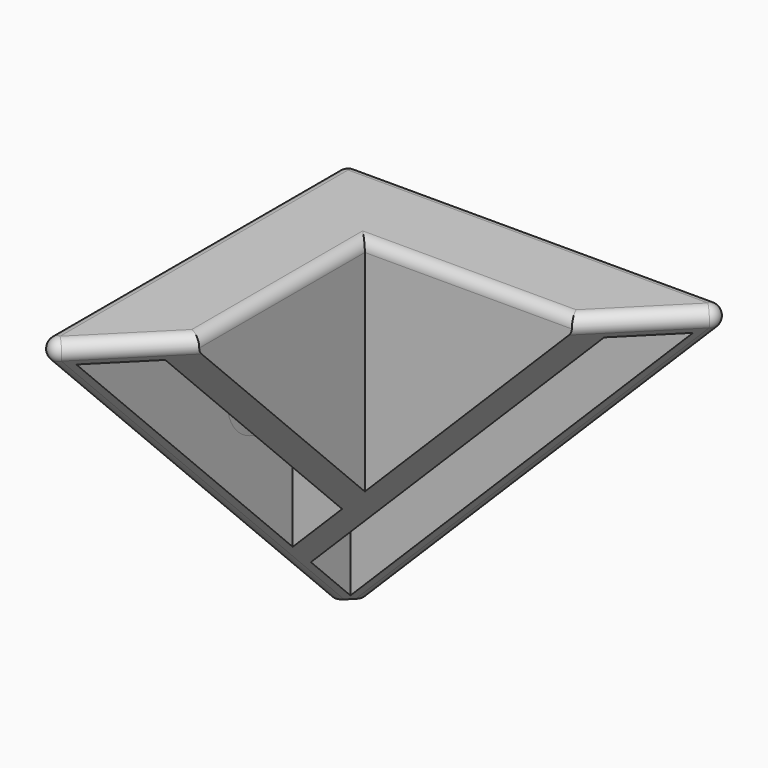
from build123d import *

# Parameters (mm, degrees)
F1_DEPTH  = 28.575
F3_R      = 38.1
F4_DEPTH  = 32.9965678842
F6_W      = 26.9748
F6_H      = 3.429
F6_W_2    = 3.429
F6_H_2    = 21.971
F7_DEPTH  = 26.9758
F14_R     = 0.762
F15_W     = 1.8396307345
F15_H     = 3.0181135691
F16_DEPTH = 26.4941772846


# Not quite as in the source:
# - a fillet or chamfer that OpenCascade refuses, or shapes differently, is made with other operations: its cross-section is extruded or revolved along the edge and cut away or added
# - a pattern or mirror of a feature is missing from the dataset's text; its kind, count and spacing are read off the source's solid


with BuildPart() as f1:
    # F0 (on Top) → F1 (new body)
    with BuildSketch(Plane.XY):
        Polygon((0, -21.971), (0, 0), (21.971, 0), (21.971, 6.604), (-6.604, 6.604), (-6.604, -21.971), align=None)
    extrude(amount=-F1_DEPTH)

    # F3 (on 3pt) → F4 (cut, through all)
    with BuildSketch(Plane(origin=(5.1223333333, -5.1223333333, -5.1223333333), x_dir=(0.4082482905, 0.8164965809, -0.4082482905), z_dir=(0.5773502692, -0.5773502692, -0.5773502692))):
        Circle(F3_R)
    extrude(amount=F4_DEPTH, mode=Mode.SUBTRACT)

    # F6 (on offset) → F7 (cut, through all)
    with BuildSketch(Plane.XY.offset(-1.6002)):
        with Locations((8.4836, 3.2893)):
            Rectangle(F6_W, F6_H)
        with Locations((-3.2893, -10.9855)):
            Rectangle(F6_W_2, F6_H_2)
    extrude(amount=-F7_DEPTH, mode=Mode.SUBTRACT)

    # F9 (on offset) → F10 (revolve)
    with BuildSketch(Plane.YZ.offset(2.6162)):
        with BuildLine():
            ThreePointArc((4.2418, -9.2202), (4.4469151823, -9.9607308906), (5.0038, -10.4902))
            Line((5.0038, -10.4902), (5.0038, -9.2202))
            Line((5.0038, -9.2202), (4.2418, -9.2202))
        make_face()
    f10 = revolve(axis=Axis((2.6162, 4.6228, -9.2202), (0, -1, 0)))

    # F10_copies: F10 across plane
    add(f10.mirror(Plane(origin=(0, 0, 0), x_dir=(0.7071067796, -0.7071067828, 0), z_dir=(-0.7071067828, -0.7071067796, 0))))

    # F13: fillet of radius 5.08 on 3 edges, made by hand

    # F13_s1 → F13_t2 (revolve)
    with BuildSketch(Plane.YZ.offset(2.6162)):
        with BuildLine():
            ThreePointArc((5.0038, -12.278765023), (4.853123865, -11.0506908258), (4.4100337662, -9.8954676025))
            ThreePointArc((4.4100337662, -9.8954676025), (4.662543942, -10.2371346569), (5.0038, -10.4902))
            Line((5.0038, -10.4902), (5.0038, -12.278765023))
        make_face()
    revolve(axis=Axis((2.6162, 5.0038, -9.2202), (0, -1, 0)))

    # F13_s3 → F13_t4 (revolve)
    with BuildSketch(Plane.XZ.offset(2.6161999777)):
        with BuildLine():
            ThreePointArc((-5.0038, -12.2787650011), (-4.8531238674, -11.0506908133), (-4.4100337753, -9.8954675976))
            ThreePointArc((-4.4100337753, -9.8954675976), (-4.6625439517, -10.237134655), (-5.0038000116, -10.4902))
            Line((-5.0038000116, -10.4902), (-5.0038, -12.2787650011))
        make_face()
    revolve(axis=Axis((-5.0038000116, -2.6161999777, -9.2202), (-1, 4.4e-09, 0)))

    # F14
    f14_edges = [f1.edges().sort_by_distance(p)[0] for p in [
        (7.6835, 6.604, 0),
        (-6.604, 6.604, -14.2875),
        (7.6835, 6.604, -14.2875),
        (-6.604, -7.6835, 0),
        (-6.604, -7.6835, -14.2875),
        (18.669, 3.302, 0),
        (7.6835, 0, 0),
        (0, -7.6835, 0),
        (-3.302, -18.669, 0),
    ]]
    fillet(f14_edges, radius=F14_R)

    # F15 (on face) → F16 (cut, through all)
    with BuildSketch(Plane(origin=(-6.604, 0, 0), x_dir=(0, -1, 0), z_dir=(-1, 0, 0))):
        with Locations((-5.6841846327, -27.2402340692)):
            Rectangle(F15_W, F15_H)
    extrude(amount=-F16_DEPTH, mode=Mode.SUBTRACT)


solid = f1.part
